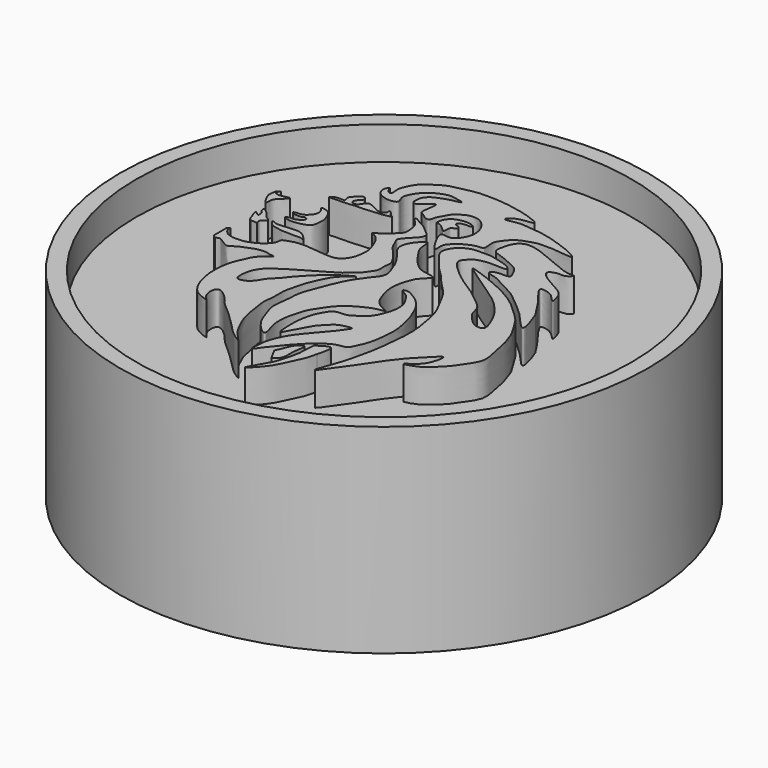
from build123d import *

# Parameters (mm, degrees)
F2_DEPTH  = 60
F3_DEPTH  = 60
F4_DEPTH  = 60
F5_DEPTH  = 60
F6_DEPTH  = 60
F7_DEPTH  = 60
F8_DEPTH  = 60
F9_DEPTH  = 60
F10_DEPTH = 60
F11_DEPTH = 60
F12_DEPTH = 60
F13_DEPTH = 60
F14_DEPTH = 60
F15_DEPTH = 60
F0_R      = 79.4315961508
F0_R_2    = 74.4995271211
F16_DEPTH = 60
F17_DEPTH = 50


with BuildPart() as f2:
    # F1 (on face) → F2 (new body)
    with BuildSketch(Plane.XY):
        with BuildLine():
            add(Edge.make_bspline(
                [(-25.1488033682, 33.7133072317), (-24.948841088, 33.6554055638), (-25.0295864981, 32.2952375615), (-22.7551749783, 31.1580490492), (-23.6359349734, 34.4213041261), (-22.5255529942, 36.8969572813), (-20.9887534088, 39.776852732), (-17.8746981156, 41.548958663), (-15.5329089333, 43.1787274213), (-11.8665002329, 43.7717071714), (-8.4590988449, 44.7027018137), (-5.1828009069, 44.8521876272), (-1.1768115878, 44.7705176008), (2.9007180169, 44.2375848697), (6.6841887942, 43.4421139413), (9.4047457297, 42.6677786162), (14.0223637788, 40.771432856), (9.0739956565, 40.5525862782), (7.7355092347, 39.919706461), (6.8017821417, 39.7666165392), (4.6771433634, 37.4517705589), (9.651774137, 38.8817918711), (11.9523997047, 38.4619543185), (15.5134078486, 38.296345935), (18.6202369187, 37.6878982564), (22.0817429014, 36.7300285599), (25.2590214422, 35.5792190237), (26.9350094416, 34.9827390019), (32.3387299286, 32.2345342215), (24.6677253907, 33.5041153846), (22.3702142175, 33.3721670882), (19.5913401559, 33.5642682328), (16.7071995749, 32.4909140871), (14.0909788157, 31.5624330143), (12.2081344098, 29.2644722909), (10.637791559, 26.9795601204), (11.7320767906, 23.2935134602), (9.3888992863, 23.5231228188), (7.0847764413, 22.6638178094), (5.3482075138, 21.7027677057), (3.7737492872, 20.2886790383), (2.2671681823, 18.7781311135), (3.3463068001, 13.6622313561), (-3.1131224014, 24.214561915), (1.5503065124, 22.2574979025), (3.4773348505, 23.9136026422), (4.8932640063, 26.3636257711), (5.0026084116, 29.0111614257), (4.2133861234, 31.4635114152), (2.2769755793, 33.8530631132), (0.0664367621, 34.6534500458), (-2.5018393163, 34.3215902544), (-3.9733032439, 33.3281410586), (-5.7722556965, 32.0548275906), (-6.5164486797, 30.1206753267), (-7.555684618, 28.8668602689), (-7.7012016356, 26.433035483), (-9.5703340628, 27.0330031457), (-10.7594975132, 28.2654632566), (-11.9803543994, 28.4486728417), (-11.6099857071, 31.2633726711), (-10.9441012767, 35.0474634302), (-13.8731895497, 32.3257538657), (-14.9203635972, 31.151310017), (-16.622592113, 31.1318908236), (-16.5655615782, 33.0655438441), (-16.2974432814, 34.6589808607), (-14.7196124342, 36.3255933191), (-12.2509273921, 37.1340369864), (-10.6075963058, 37.8476618897), (-6.1226589069, 38.5279588204), (-9.9184187928, 39.2690962757), (-11.7829877097, 39.625900886), (-14.3398408927, 38.8250281602), (-16.4524932331, 37.5812630174), (-18.0683920322, 36.2192233402), (-19.4918002513, 33.9877151645), (-20.4148396915, 31.7160870717), (-18.5406189783, 29.1629240945), (-21.6869946154, 28.5886242761), (-23.8178789386, 29.2487292901), (-25.4085790801, 30.1169536255), (-26.4301310689, 32.4230550039), (-25.3572237428, 33.7736580503), (-25.1488033682, 33.7133072317)],
                knots=[0, 0, 0, 0, 0.0088010468, 0.01825747, 0.0300012191, 0.0431291225, 0.0568876526, 0.0712947967, 0.0843234785, 0.0990386418, 0.1135859474, 0.1274974267, 0.142923044, 0.1587382972, 0.1736292931, 0.1878326308, 0.2009766337, 0.2146363917, 0.2246553918, 0.2324142696, 0.2423432307, 0.2567604877, 0.2697582943, 0.2839242077, 0.29780578, 0.3125802409, 0.3263527799, 0.3380840838, 0.3520524286, 0.3691845538, 0.3824486865, 0.3947658058, 0.4083026863, 0.4210882833, 0.4341529226, 0.4470600717, 0.460318558, 0.4701240818, 0.4824347944, 0.4933370912, 0.5043941458, 0.5160546105, 0.5273804796, 0.5482747699, 0.5600336456, 0.5721435882, 0.5849909532, 0.5973202677, 0.6096733329, 0.6229435032, 0.6346210947, 0.6466958716, 0.6570142102, 0.6682888819, 0.6791909485, 0.6892798089, 0.6999278038, 0.7090859349, 0.7193906789, 0.7266444046, 0.7395084249, 0.7518234496, 0.7643086169, 0.7748137274, 0.7831375363, 0.7928370108, 0.8028110507, 0.8141778144, 0.8262877958, 0.8378671653, 0.8508323451, 0.8622235016, 0.8738485587, 0.8861192779, 0.8982292241, 0.9093881265, 0.9219095693, 0.9337973758, 0.9452912312, 0.9568705946, 0.9687588458, 0.9789672473, 0.9908266826, 1, 1, 1, 1], degree=3))
        make_face()
    extrude(amount=F2_DEPTH)


with BuildPart() as f3:
    # F1 (on face) → F3 (new body)
    with BuildSketch(Plane.XY):
        with BuildLine():
            add(Edge.make_bspline(
                [(-26.945585385, 26.3207778335), (-26.5811278754, 26.1919596539), (-25.9021475482, 25.1956940165), (-27.1545322644, 24.3076704164), (-27.7499431243, 23.494602771), (-27.7574333029, 22.2275042374), (-25.897747523, 22.0822792358), (-25.2380605037, 23.4164596333), (-24.2446991532, 24.791559816), (-22.654971193, 24.0563709455), (-20.8721222009, 23.2639980649), (-19.5544966211, 22.4326581284), (-17.5785439162, 23.2834334669), (-18.3095323689, 24.7421037011), (-16.8497931436, 24.0017664095), (-16.7134374099, 22.9181613345), (-15.0603218715, 22.6683654735), (-17.6513601518, 22.0278243921), (-19.5107603166, 21.9286761464), (-21.411838687, 21.7967317051), (-23.4247126983, 21.4454191784), (-25.8274115732, 21.6250141179), (-27.7736671913, 21.2576014296), (-29.5985925328, 21.1885655512), (-31.475130181, 21.3117028241), (-34.3827292896, 20.8634787724), (-31.7377232386, 22.633539097), (-28.9241161492, 21.7104302415), (-30.2136237715, 23.6000988053), (-29.1775773466, 24.8158836205), (-28.1456552657, 25.9685139895), (-27.3010351747, 26.4464122178), (-26.945585385, 26.3207778335)],
                knots=[0, 0, 0, 0, 0.029621162, 0.0602606581, 0.0878346733, 0.114159912, 0.145918635, 0.178271441, 0.2105854405, 0.2435742709, 0.2818298618, 0.3152731713, 0.3499786591, 0.3751276802, 0.4016893464, 0.4305616795, 0.4548520971, 0.4904756287, 0.5303717086, 0.5667593396, 0.6053166578, 0.6470565607, 0.6849271688, 0.7205384141, 0.7603358376, 0.7959315555, 0.8338938186, 0.873661734, 0.9039971078, 0.9365658208, 0.9711109374, 1, 1, 1, 1], degree=3))
        make_face()
    extrude(amount=F3_DEPTH)


with BuildPart() as f4:
    # F1 (on face) → F4 (new body)
    with BuildSketch(Plane.XY):
        with BuildLine():
            add(Edge.make_bspline(
                [(-41.7717136443, -5.5398973636), (-41.812882174, -5.8481698397), (-41.900913535, -6.5073540721), (-41.1781574572, -7.5221923251), (-40.3650623179, -8.3312059894), (-39.5128472879, -8.6372278935), (-38.2526650737, -9.0186086654), (-37.1477285954, -8.9206808049), (-35.7296906683, -8.9229396647), (-34.5576650094, -8.7253272454), (-33.2534097973, -8.2178484871), (-32.019836988, -7.6898016339), (-30.6539944827, -6.8020483209), (-29.5403590759, -5.7476969367), (-28.5482811, -4.3460828042), (-28.8079652144, -2.7393990339), (-27.0064684474, -2.3854852368), (-25.7897787275, -1.8195429094), (-24.2005614178, -1.5944809385), (-22.5584335536, -1.5454733348), (-21.0198860982, -1.6673648427), (-19.3801408161, -1.8562747679), (-17.8724149763, -1.8866949794), (-16.5955273937, -2.1853103978), (-15.0944833944, -2.2375183906), (-13.6987284549, -2.3214296878), (-12.4195594167, -1.9381450275), (-11.0800652344, -1.0484762075), (-10.0296859586, 0.679056702), (-9.5919889509, 2.0539459798), (-9.3615036071, 3.8522474844), (-9.2287679772, 5.4900772478), (-9.7081055721, 7.3552492356), (-10.3886506746, 9.1952918081), (-11.1059511983, 10.8186935734), (-12.3357157318, 12.3516107548), (-13.5188638139, 12.9202228105), (-14.1151761636, 13.2068060338)],
                knots=[0, 0, 0, 0, 0.0226010476, 0.0483282012, 0.0732757833, 0.0955379345, 0.1220339325, 0.1470203337, 0.1747103132, 0.2004493041, 0.227908869, 0.2552804598, 0.2849714154, 0.3143497788, 0.3446015362, 0.3714995697, 0.4004560514, 0.4283986079, 0.4577769801, 0.4879190496, 0.5171292411, 0.5473299531, 0.5760514088, 0.6028558433, 0.6315773079, 0.6592578181, 0.6858933962, 0.7154604959, 0.7484178018, 0.7768371052, 0.8080658597, 0.8382079398, 0.8705581331, 0.9035154357, 0.9347771966, 0.9671273919, 1, 1, 1, 1], degree=3))
            Line((-41.7717136443, -5.5398973636), (-42.4412414432, -6.312427111))
            Line((-42.4412414432, -6.312427111), (-42.4412414432, -10.8445966616))
            add(Edge.make_bspline(
                [(-42.4412414432, -10.8445966616), (-42.3518233963, -10.9601905606), (-42.2624053495, -11.0757844595), (-42.1685176486, -11.1777507043)],
                knots=[0, 0, 0, 0, 0.0071487722, 0.0071487722, 0.0071487722, 0.0071487722], degree=3))
            Line((-42.1685176486, -11.1777507043), (-41.6172109544, -11.5141225979))
            add(Edge.make_bspline(
                [(-41.6172109544, -11.5141225979), (-41.2739568617, -11.5529146812), (-40.5164359526, -11.1174211196), (-39.939617102, -11.4287726818), (-38.5882424276, -12.1381249694), (-36.8538881302, -13.5066791968), (-35.2969900432, -12.2715700906), (-34.1373228627, -11.5753695582), (-31.8539806603, -10.7248807675), (-30.0471463451, -9.9729712348), (-27.2249383164, -9.7223761824), (-26.1800156346, -10.4058344081), (-23.8508093777, -10.1587301465), (-27.812550286, -12.6035494239), (-29.180312977, -15.5258197947), (-30.5844211722, -18.8364875768), (-31.2745911855, -21.6552347309), (-31.398421323, -25.645852678), (-31.0543413286, -28.5636241287), (-29.9953288887, -32.4181815819), (-28.4499579521, -34.7867259671), (-26.8917633836, -36.4207970984), (-22.4800073499, -38.0152544708), (-24.4379324911, -36.6925787292), (-25.1809842613, -35.069793224), (-25.4038326659, -33.248258278), (-24.5324112909, -30.6659563525), (-20.2835539037, -34.1763577811), (-18.790274815, -36.6676925534), (-16.2776501448, -38.467778442), (-13.3398116362, -41.3645848972), (-10.3799188446, -44.1175352927), (-8.1093470247, -46.9412037763), (-4.7698938059, -49.0398547747), (-4.6388213523, -48.9560291171)],
                knots=[0.0195308088, 0.0195308088, 0.0195308088, 0.0195308088, 0.0395165176, 0.0540412535, 0.0776082575, 0.1044403461, 0.1288503292, 0.1515243185, 0.1804790807, 0.2080591077, 0.2388047116, 0.2611253909, 0.2813945091, 0.3151607814, 0.3515490656, 0.3867193244, 0.419334208, 0.4566014451, 0.4897577827, 0.5273175728, 0.5584787467, 0.5892243548, 0.6233580824, 0.6431699724, 0.6695429055, 0.6957509905, 0.720370143, 0.7602568507, 0.7942585309, 0.8266566241, 0.8652890023, 0.9030538629, 0.9420116676, 0.9771089014, 0.9771089014, 0.9771089014, 0.9771089014], degree=3))
            add(Edge.make_bspline(
                [(-4.6388213523, -48.9560291171), (-4.9352998348, -48.6181442496), (-5.2317783172, -48.2802593821), (-5.6173582561, -47.8744879365)],
                knots=[0, 0, 0, 0, 0.0158560937, 0.0158560937, 0.0158560937, 0.0158560937], degree=3))
            add(Edge.make_bspline(
                [(-5.6173582561, -47.8744879365), (-6.13474356, -47.3300089284), (-7.548026456, -45.9398789902), (-8.9315413686, -43.2228054554), (-10.5436119615, -39.9309888811), (-11.3712116442, -36.3589792043), (-11.8973772942, -33.0674972474), (-12.4014600508, -29.8824723696), (-11.7468911414, -26.7704839257), (-11.993439657, -23.4515833025), (-11.6909591902, -21.3795341391), (-10.9799097981, -18.5794695303), (-10.3069577448, -16.3046017593), (-9.2280499592, -13.8182916861), (-8.0760118861, -11.3256808911), (-6.6203654418, -8.9371992375), (-1.7089230724, -5.342087689), (-6.1912461596, -7.8936037937), (-7.942417065, -8.9973623835), (-9.8992416077, -10.9354922771), (-11.7021927255, -12.2806854067), (-12.845209808, -13.7144930258), (-14.8131809385, -15.5870056396), (-16.1569615177, -17.535083997), (-17.4727506994, -18.9539412911), (-18.7450287181, -19.9461027976), (-19.6581344178, -21.6425690566), (-20.910821323, -23.5140413465), (-22.6155281543, -24.6245194996), (-24.6213957754, -24.7646790892), (-24.9895903234, -23.2788042047), (-24.7939524692, -20.5410899606), (-23.9348150765, -18.4398883996), (-22.3816862999, -16.1984506269), (-19.9266940951, -14.7369965943), (-18.0056654028, -13.4090371178), (-16.0930830842, -12.2615334721), (-14.0016017074, -11.2367777297), (-12.1232802741, -9.9159570246), (-9.2286573318, -8.348466506), (-6.8676607355, -6.9464720931), (-5.3930549939, -5.5967884098), (-3.3064302904, -3.8569690441), (-2.193528738, -2.1649292562), (-1.0010126621, -0.4512955562), (-1.466167431, 1.9274365828), (-0.9268812345, 3.716208247), (-1.643877149, 5.1980681997), (-2.1296237756, 6.0366131533), (-2.4242375512, 6.4600519836)],
                knots=[0.0158560937, 0.0158560937, 0.0158560937, 0.0158560937, 0.0371323817, 0.060218382, 0.0853556994, 0.1105165445, 0.1345271615, 0.1578543777, 0.1813702144, 0.2050197665, 0.2241688148, 0.2461795058, 0.2666340445, 0.2881199778, 0.3093962662, 0.3334182674, 0.3586284508, 0.3808198369, 0.4019889386, 0.4232652291, 0.4428666193, 0.4605902908, 0.4821473833, 0.5025765464, 0.5206506722, 0.5370825703, 0.5551800108, 0.5748542534, 0.5936898225, 0.6105447794, 0.6250713915, 0.6467937641, 0.6667689254, 0.6881306205, 0.7102713498, 0.7303665647, 0.7499154225, 0.7697456307, 0.7897207953, 0.8136498657, 0.8353414112, 0.8539609946, 0.875377061, 0.8942214699, 0.9125919059, 0.9325794234, 0.9502390418, 0.966485755, 0.9825739497, 0.9825739497, 0.9825739497, 0.9825739497], degree=3))
            add(Edge.make_bspline(
                [(-3.1750648823, 7.4446975933), (-2.9115332904, 7.1126724104), (-2.6678854208, 6.786362197), (-2.4242375512, 6.4600519836)],
                knots=[0.9672997896, 0.9672997896, 0.9672997896, 0.9672997896, 1, 1, 1, 1], degree=3))
            add(Edge.make_bspline(
                [(-3.1750648823, 7.4446975933), (-3.2842875071, 7.5798804629), (-3.3950326538, 7.7152422973), (-3.5057778005, 7.8506041318)],
                knots=[0.9949376131, 0.9949376131, 0.9949376131, 0.9949376131, 1, 1, 1, 1], degree=3))
            add(Edge.make_bspline(
                [(-10.8190523461, 15.4728898779), (-10.3854274198, 15.9336787565), (-9.5163377594, 16.8572115744), (-7.9802574199, 18.2941033182), (-8.3260002082, 20.4083149948), (-8.4757768683, 22.1852635368), (-9.7512213256, 24.0889997591), (-10.895274758, 24.7182313128), (-10.7579373208, 25.8043581105), (-9.0650849821, 24.457150277), (-7.5303322035, 23.8564050674), (-6.0899522703, 22.7885843373), (-4.9157662853, 21.7113410883), (-3.0425480104, 20.3796482699), (-4.1710010675, 18.0976920702), (-5.8586829505, 16.777319173), (-6.6032379897, 15.7692465224), (-7.4062633733, 14.791681699), (-7.6077682259, 14.1723810275), (-7.1992699425, 13.2583242463), (-6.5296983611, 11.9137837642), (-5.8845376145, 10.4732748357), (-4.8420733277, 9.3388785602), (-3.9296511659, 8.3564771008), (-3.5057778005, 7.8506041318)],
                knots=[0, 0, 0, 0, 0.0480714388, 0.0963468378, 0.1447484497, 0.1916578957, 0.2433048134, 0.2818038524, 0.3068780104, 0.3517429601, 0.3990073719, 0.4441227469, 0.4889877125, 0.537093329, 0.5876362656, 0.6387792572, 0.6779119067, 0.7160563974, 0.7425690758, 0.775907016, 0.8188890711, 0.8621906045, 0.9050766017, 0.9540786737, 0.9540786737, 0.9540786737, 0.9540786737], degree=3))
            Line((-10.8190523461, 15.4728898779), (-12.4156121165, 14.3913496286))
            Line((-12.4156121165, 14.3913496286), (-14.1151761636, 13.2068060338))
        make_face()
    extrude(amount=F4_DEPTH)


with BuildPart() as f5:
    # F1 (on face) → F5 (new body)
    with BuildSketch(Plane.XY):
        with BuildLine():
            add(Edge.make_bspline(
                [(-1.0437119054, 17.6707785577), (-0.6680510269, 17.5281639166), (-0.7167650455, 15.2486465781), (-0.1383137822, 13.1744180567), (1.4633481849, 10.8526251062), (3.1842207352, 8.5119758865), (4.9045450056, 6.7976612166), (7.1274400052, 5.2019533428), (12.4785569794, 5.0404475679), (8.8068904067, 2.095643908), (7.8800533811, 0.092999726), (6.9423578386, -2.7867882957), (6.6287030782, -5.4702540952), (6.9569071786, -8.0680856615), (7.8153266384, -10.6998051683), (8.756228694, -13.1108677491), (11.0125471571, -14.939419708), (14.0214915667, -15.8635478322), (10.7524809013, -16.2119972845), (8.7107193825, -17.0039249448), (6.2489918759, -18.2535355851), (3.5314768148, -20.0089368628), (1.3909330893, -22.3069682992), (0.0560761569, -24.6098040978), (-1.5814909932, -26.726094315), (-2.3159028616, -29.5048403305), (-3.1679217561, -32.3136394185), (-3.3420829586, -35.1384357614), (-3.3290705866, -37.5730381049), (-0.8084833727, -44.3143001347), (-6.596131401, -38.7794677774), (-7.6332647839, -35.1666610179), (-9.5971218339, -30.6324477031), (-8.4865291526, -25.8276229918), (-8.6196646513, -21.382188177), (-6.8158572369, -17.0904387558), (-5.3665305092, -13.0669644448), (-3.1739157096, -8.2219797981), (-0.1030258548, -4.2247765634), (2.1151935011, -1.6009824249), (0.9362872124, 1.8692482935), (0.0377103781, 3.9900265033), (-0.9832666615, 6.0099020432), (-2.4965594418, 8.0176422967), (-3.9154209394, 9.6410443313), (-5.0477323701, 11.748995492), (-4.2503586834, 14.4595533475), (-3.0391121083, 16.0744532453), (-1.4262579955, 17.8160070775), (-1.0437119054, 17.6707785577)],
                knots=[0, 0, 0, 0, 0.0180662574, 0.0370243927, 0.0572922299, 0.0781994976, 0.0968854477, 0.1180022755, 0.1410798269, 0.1619870944, 0.1814118083, 0.2022720423, 0.2223951554, 0.2420617116, 0.2623294907, 0.2817267352, 0.3033696958, 0.3200464418, 0.3374137738, 0.3568024159, 0.3768221173, 0.3988895748, 0.4204704133, 0.4403559629, 0.4601258519, 0.4807435185, 0.5018046219, 0.5216767991, 0.5426840016, 0.568043086, 0.5947742813, 0.6206060917, 0.6468109106, 0.6736301198, 0.6993468146, 0.7253083304, 0.7506873126, 0.7789229723, 0.8065436837, 0.8282051818, 0.8504312216, 0.8692606168, 0.8874684285, 0.9067849697, 0.9248299152, 0.9431665618, 0.9627584908, 0.9816026194, 1, 1, 1, 1], degree=3))
        make_face()
    extrude(amount=F5_DEPTH)


with BuildPart() as f6:
    # F1 (on face) → F6 (new body)
    with BuildSketch(Plane.XY):
        with BuildLine():
            add(Edge.make_bspline(
                [(0.4940500367, -50.237737596), (0.2347112404, -50.1195504862), (0.5103066985, -47.4874990383), (0.6769040843, -45.0440917932), (2.1339693914, -41.387622137), (3.7050160139, -38.788399872), (5.5412466048, -36.4827920712), (7.5080406202, -34.059883027), (9.1278798858, -32.2046935016), (10.817283103, -30.3183952304), (11.7871385117, -28.756592706), (12.913744567, -27.2920623088), (10.8645915202, -27.6372803151), (9.1758834595, -28.045283632), (7.7349563595, -28.8341818338), (6.7234678053, -30.0781462797), (4.937185354, -31.5497243064), (4.0600879869, -33.4080920458), (2.9510748569, -35.3481109623), (2.0395521703, -37.0697354357), (0.1941023116, -40.8101834603), (-0.0407907522, -36.3089590013), (-0.0862577122, -32.928061746), (0.2851370233, -30.5971327924), (0.8636496911, -27.907516707), (2.0920215601, -25.5912182347), (3.6020632392, -22.9439175481), (7.1936462029, -23.4366390418), (9.3826788863, -21.8747289588), (11.6009228324, -20.3955708455), (12.9255803466, -18.5621536991), (13.9308463686, -15.8953019128), (14.4420616775, -14.0800720035), (14.5271562157, -11.8264624082), (14.101712928, -9.6678742439), (12.7191991714, -7.8264112035), (12.0383492387, -6.4096361583), (8.8970202336, -5.0291598162), (10.875153716, -4.505029197), (12.2033139347, -5.129919921), (13.6829661571, -6.0354938103), (15.3539093605, -7.1813244889), (17.1367785085, -9.3188485096), (18.1008405424, -11.0387425305), (19.0196753174, -13.1890438649), (19.741040379, -15.0893606472), (20.3382996294, -17.7424175921), (21.0256114221, -20.5509737958), (21.0761135855, -23.1828525784), (20.8751044174, -26.0087300637), (20.614340675, -28.0506451612), (20.2424546588, -30.1395741867), (19.4532606788, -32.5298353778), (18.2661964925, -34.664102346), (17.8276740631, -36.0436387849), (14.7465090721, -36.1943572681), (12.7880443546, -37.3293463405), (10.1399092464, -38.9882995494), (8.8930488795, -40.4857162659), (6.7513341101, -42.4857538759), (5.3258674891, -44.3866293902), (3.956265061, -46.164528699), (2.5469205402, -47.6785213598), (1.6248592215, -49.0790783624), (0.6928079738, -50.3283165086), (0.4940500367, -50.237737596)],
                knots=[0, 0, 0, 0, 0.016092581, 0.0339180945, 0.0542546768, 0.0726261625, 0.0905454831, 0.1089768296, 0.125528269, 0.1420012813, 0.1569421521, 0.1681094906, 0.1804153048, 0.1950621104, 0.2080806766, 0.2212961181, 0.2370405629, 0.2521013168, 0.2673254649, 0.2833442438, 0.300080553, 0.3175782129, 0.3381229247, 0.3540067764, 0.3710886691, 0.388287161, 0.4054284384, 0.4241330749, 0.4411742212, 0.4580394929, 0.4737808842, 0.49126021, 0.5057400352, 0.5212046687, 0.5367470273, 0.552166403, 0.5661436695, 0.582433472, 0.5931432897, 0.6062331914, 0.6198651472, 0.6348545476, 0.6521589106, 0.6670375318, 0.6827840063, 0.6977604311, 0.7149550262, 0.7327651008, 0.7498254562, 0.7673580245, 0.7823521462, 0.7974302904, 0.8142290104, 0.8305224727, 0.8421328097, 0.8594126185, 0.8757644806, 0.8938490556, 0.9086719618, 0.926354973, 0.9426731525, 0.9582899971, 0.973134778, 0.9876666035, 1, 1, 1, 1], degree=3))
        make_face()
    extrude(amount=F6_DEPTH)


with BuildPart() as f7:
    # F1 (on face) → F7 (new body)
    with BuildSketch(Plane.XY):
        with BuildLine():
            add(Edge.make_bspline(
                [(18.8469719142, -49.53160882), (19.0719934178, -49.7806545768), (22.1820032384, -45.1675211505), (24.9498112967, -41.4884438044), (28.2823518318, -36.2176271983), (32.1522982817, -31.1392206388), (35.0094858383, -28.5958512011), (39.1708604148, -23.9237279851), (37.8900953309, -29.5209605135), (36.2269444405, -32.0675609996), (31.2969069001, -35.0225041773), (37.9577931773, -32.9049060194), (39.8493853557, -30.7644924399), (42.5022304615, -28.3358545822), (44.2052156674, -25.5412026302), (47.4071728821, -21.2312810717), (46.1274634213, -16.6364442877), (45.4475723483, -11.749863183), (43.682085657, -6.5668487602), (41.7652391551, -3.4741507812), (39.6282176401, 0.1751620257), (36.822389871, 2.5221662407), (33.673143652, 5.7327524555), (29.3913591405, 8.4482157029), (25.156195807, 10.5358196796), (21.5820066085, 12.0528026369), (13.1661169107, 15.0802421545), (19.0660731609, 11.5092591014), (21.7037620816, 9.3272432684), (27.1985330921, 5.9511986834), (30.89814968, 2.9897342932), (33.9961501286, -0.7728069078), (35.6436677508, -4.0979926535), (37.3656798254, -8.4616665489), (34.6283021517, -8.7676373231), (32.6239250148, -7.5852406186), (31.2234280381, -5.9426974036), (29.4838217628, -3.9510923182), (29.2524809999, -0.8094724846), (26.0012073144, 1.6927222035), (22.8203343946, 4.3843027436), (18.0123310614, 7.2343368085), (14.5365009944, 9.9977470824), (9.7149973199, 14.3819314201), (11.6389380182, 16.4681916567), (12.9552353036, 17.7816594832), (15.0201346783, 18.2623102132), (17.0260002138, 18.6956982605), (23.5203177194, 18.0844792438), (20.4331307224, 20.2287318766), (17.6651520408, 20.909910287), (14.7226763173, 21.7472413513), (11.8052194672, 21.5225727179), (9.3014093082, 21.6154325262), (6.8987181979, 20.4256415602), (5.2647809323, 18.9434437302), (3.7305111876, 15.7010228061), (6.6289901989, 12.6125540069), (8.8156005327, 9.298601563), (11.7182351492, 7.0041244456), (14.4797531628, 3.1693747907), (18.067790695, 0.1613400375), (19.8224203572, -3.5763257464), (22.8492347556, -8.5650387364), (23.7374692041, -13.9485850872), (24.609976637, -18.6264458729), (24.528291617, -23.4322570166), (23.9885820292, -28.2590560778), (23.446831198, -33.2800633714), (22.1636596445, -37.9229475354), (21.7820609301, -41.3542064841), (18.5537031421, -49.2070294259), (18.8469719142, -49.53160882)],
                knots=[0, 0, 0, 0, 0.0154284311, 0.0323573138, 0.0500648858, 0.0679112112, 0.0831526279, 0.0972034724, 0.1102551915, 0.1246952977, 0.1371758065, 0.1520377671, 0.1653430021, 0.1783630905, 0.1915572404, 0.2075437404, 0.2226706924, 0.2387780105, 0.2553658997, 0.2691293972, 0.2835812948, 0.2972431359, 0.3123542472, 0.3285612449, 0.3436932534, 0.3594025029, 0.3763821589, 0.3900377325, 0.4048183161, 0.4225952803, 0.4384816937, 0.4538957926, 0.4684037771, 0.4822240353, 0.4918099048, 0.5027240925, 0.5132565902, 0.5246458166, 0.5368827435, 0.550908259, 0.5657881969, 0.5823957212, 0.5983693444, 0.6152724437, 0.6255622938, 0.6353924889, 0.6452112731, 0.6566597958, 0.6721487313, 0.6818639569, 0.694735138, 0.7071617154, 0.7193268082, 0.7306219465, 0.7420160056, 0.752745552, 0.7652098764, 0.7792796245, 0.7936538272, 0.807301657, 0.8228386421, 0.8381623151, 0.8526245498, 0.8698046014, 0.8865364521, 0.9021037081, 0.9176819809, 0.9334847207, 0.9496973721, 0.9647836761, 0.979892246, 1, 1, 1, 1], degree=3))
        make_face()
    extrude(amount=F7_DEPTH)


with BuildPart() as f8:
    # F1 (on face) → F8 (new body)
    with BuildSketch(Plane.XY):
        with BuildLine():
            add(Edge.make_bspline(
                [(10.9271435067, -39.9931296706), (12.5184241223, -38.9472879149), (15.8009471323, -36.7899062473), (14.7590611641, -40.849683481), (14.2222540453, -42.9413877428)],
                knots=[0, 0, 0, 0, 0.4847736362, 1, 1, 1, 1], degree=3))
            add(Edge.make_bspline(
                [(10.9271435067, -39.9931296706), (10.9023231736, -41.0342740665), (10.8508065563, -43.1952538249), (10.4849553834, -46.6381873854), (9.0924118884, -51.6404795111), (8.0501965506, -53.6280423898), (3.4148855505, -61.1908405175), (8.7959842228, -55.3563999889), (10.2086672648, -53.0563340807), (11.6766764644, -49.8775775908), (13.3904573107, -46.5748678482), (13.9454153453, -44.1506830756), (14.2222540453, -42.9413877428)],
                knots=[0, 0, 0, 0, 0.0903517968, 0.1875324929, 0.2998290507, 0.3902277539, 0.5079314891, 0.6153417282, 0.7098124994, 0.8024437195, 0.9014498025, 1, 1, 1, 1], degree=3))
        make_face()
    extrude(amount=F8_DEPTH)


with BuildPart() as f9:
    # F1 (on face) → F9 (new body)
    with BuildSketch(Plane.XY):
        with BuildLine():
            add(Edge.make_bspline(
                [(7.1117510088, -51.2658767402), (7.6545782942, -50.8629127925), (8.7366697364, -50.05962996), (9.3143626448, -47.9651218624), (8.8754641497, -45.2667386156), (10.2592459537, -40.5686658048), (6.9777213692, -42.9193336391), (6.3440442839, -45.421277968), (5.5772985706, -46.9805111166), (5.2040554583, -47.7395281196)],
                knots=[0, 0, 0, 0, 0.1254672787, 0.2501109879, 0.4083132923, 0.5710366016, 0.7071200236, 0.857429351, 1, 1, 1, 1], degree=3))
            Line((5.2040554583, -47.7395281196), (7.1117510088, -51.2658767402))
        make_face()
    extrude(amount=F9_DEPTH)


with BuildPart() as f10:
    # F1 (on face) → F10 (new body)
    with BuildSketch(Plane.XY):
        with BuildLine():
            add(Edge.make_bspline(
                [(-31.4861834049, 15.7587900758), (-31.5759823818, 15.6118638231), (-30.79941485, 14.9140694565), (-30.3727654897, 13.9926087382), (-30.4154143053, 13.2584727133), (-30.6098150818, 12.2179853039), (-31.3314528041, 11.5234377386), (-31.8224715842, 10.7800885518), (-33.1304939599, 10.1930750641), (-34.152079337, 10.2618399416), (-35.7289554747, 9.9322818776), (-34.4641956519, 9.2467718038), (-33.5095970152, 9.2281297584), (-32.2867779063, 9.1214282455), (-31.5712395107, 9.8346093035), (-30.5024696149, 9.1775369099), (-30.748730721, 8.4259791261), (-31.656195028, 7.7679527372), (-33.0248260377, 7.0703790325), (-34.1813670012, 7.4619656113), (-35.5518656112, 6.6543599242), (-34.2934846772, 6.2581835834), (-32.7322832935, 5.9465531681), (-30.7183164114, 6.2609234504), (-28.8218630005, 6.7044202266), (-27.3171139766, 7.7703211707), (-27.2920349986, 9.4193861021), (-26.9903761949, 11.3276526021), (-27.5965299708, 12.777464978), (-28.1954108431, 14.272467911), (-29.3590579455, 15.6405045875), (-31.363965785, 15.9587586894), (-31.4861834049, 15.7587900758)],
                knots=[0, 0, 0, 0, 0.0297113266, 0.0610493523, 0.0862312126, 0.1164205144, 0.1459019463, 0.1740941202, 0.2084567041, 0.2413162573, 0.2717665383, 0.2995576028, 0.3309976102, 0.3630540712, 0.3911509081, 0.4203841521, 0.4437379248, 0.4754685834, 0.5117414545, 0.5452708252, 0.5756303936, 0.6024886166, 0.641664581, 0.6843144802, 0.7264918675, 0.7648621025, 0.8021948842, 0.843547735, 0.8806134367, 0.9179943702, 0.9595624834, 1, 1, 1, 1], degree=3))
        make_face()
    extrude(amount=F10_DEPTH)


with BuildPart() as f11:
    # F1 (on face) → F11 (new body)
    with BuildSketch(Plane.XY):
        with BuildLine():
            add(Edge.make_bspline(
                [(-44.0419688821, 16.368214041), (-44.0474841029, 16.424146657), (-44.7609867627, 15.9447441113), (-45.0799864737, 15.4089406691), (-45.243709492, 14.2780405544), (-45.3665635445, 13.2562600458), (-44.8869474236, 12.1427661002), (-44.6031998588, 11.4911866606), (-43.1932955061, 9.0931997759), (-43.1361128154, 10.6230270288), (-43.2056795038, 11.4124557877), (-42.8111420605, 12.2858205783), (-42.3245007432, 12.87806605), (-41.7150023774, 13.4820409751), (-41.1190168508, 13.8438687635), (-40.8430500091, 14.4467130017), (-39.8854828782, 15.1624469282), (-41.2243466108, 15.0178182472), (-42.1021515056, 14.7491191765), (-43.3529566282, 14.5382259461), (-44.2364614946, 14.7980531112), (-45.0532860233, 15.2966460716), (-44.0347551067, 16.2950555325), (-44.0419688821, 16.368214041)],
                knots=[0, 0, 0, 0, 0.041186125, 0.0837173187, 0.1351462678, 0.1860837788, 0.2375224576, 0.2856962306, 0.3553821942, 0.3988275644, 0.4463692659, 0.4930130755, 0.5367058855, 0.5822404606, 0.6223519232, 0.6646792967, 0.7068701433, 0.7517234337, 0.8033348098, 0.857675504, 0.9060266167, 0.9461295449, 1, 1, 1, 1], degree=3))
        make_face()
    extrude(amount=F11_DEPTH)


with BuildPart() as f12:
    # F1 (on face) → F12 (new body)
    with BuildSketch(Plane.XY):
        with BuildLine():
            Line((-40.5653752387, 0.5335501046), (-38.5018847883, 0.3714756167))
            add(Edge.make_bspline(
                [(-38.5018847883, 0.3714756167), (-38.5327005102, 0.520637011), (-38.5983048527, 0.8381903433), (-38.7674243005, 1.4708310845), (-38.617744571, 1.7459340772), (-38.3692407103, 2.0912364817), (-37.9314490014, 2.4158264954), (-36.9564980841, 3.0507527476), (-38.1160675037, 3.7283551949), (-38.8910003209, 4.270416645), (-39.5349852274, 5.3435032996), (-40.2015723412, 6.0565778491), (-40.9414152841, 6.5248978306), (-41.7435403594, 7.3689966204), (-41.7495017284, 5.8127483018), (-40.7469003387, 5.3213794614), (-40.8175417859, 4.2427247165), (-40.5967456313, 3.4197020679), (-41.5911528233, 4.1431797334), (-42.2589226664, 4.7846825267), (-42.1768148732, 3.6059718953), (-41.7327854217, 2.768480731), (-41.4491487726, 2.0607382575), (-41.2067531698, 1.0203134354), (-40.7692566878, 0.6882826085), (-40.5653752387, 0.5335501046)],
                knots=[0, 0, 0, 0, 0.0342475272, 0.0729103964, 0.0993682573, 0.1299400484, 0.1681526624, 0.2126740754, 0.2608511556, 0.3108596717, 0.3646098667, 0.4125950875, 0.4607405807, 0.5019450624, 0.5503232479, 0.6003205177, 0.6503326618, 0.6845759583, 0.7322681427, 0.7716100505, 0.8150144776, 0.8646615494, 0.9075708081, 0.9569262877, 1, 1, 1, 1], degree=3))
        make_face()
    extrude(amount=F12_DEPTH)


with BuildPart() as f13:
    # F1 (on face) → F13 (new body)
    with BuildSketch(Plane.XY):
        with BuildLine():
            add(Edge.make_bspline(
                [(-36.1724644899, 3.3190429676), (-36.1044100287, 3.4608933082), (-34.9332309581, 2.8144857174), (-33.6255644538, 2.8092829529), (-32.119794366, 2.995036459), (-30.5104220523, 2.9579475657), (-28.9213725113, 3.262059871), (-27.7641924258, 3.1005487707), (-26.5387503759, 2.4917151145), (-25.7773310297, 1.7778302718), (-25.2375014524, 1.2237177743), (-24.1081016589, 0.1541045588), (-26.0093205422, 0.9943966541), (-27.052948609, 0.7422322923), (-28.750985331, 0.8499276179), (-30.0390247069, 0.9250698369), (-31.2596527986, 0.8228241351), (-32.7113013121, 1.1495779049), (-34.0095720812, 1.4626123959), (-35.0031527009, 1.5037143674), (-36.2605231812, 3.1354965092), (-36.1724644899, 3.3190429676)],
                knots=[0, 0, 0, 0, 0.0491147433, 0.1051400747, 0.1610705449, 0.2199624616, 0.2780020591, 0.3275094725, 0.3808094485, 0.4269475752, 0.4712068093, 0.5136651527, 0.5660686552, 0.6176350889, 0.6765107173, 0.7291934608, 0.7796115905, 0.8359370279, 0.8880845161, 0.9364482513, 1, 1, 1, 1], degree=3))
        make_face()
    extrude(amount=F13_DEPTH)


with BuildPart() as f14:
    # F1 (on face) → F14 (new body)
    with BuildSketch(Plane.XY):
        with BuildLine():
            add(Edge.make_bspline(
                [(14.2801599577, 26.5449956059), (14.4576997253, 27.3012161962), (14.8014456807, 28.7653826348), (15.9049990116, 30.5684825814), (18.0360365526, 31.7161839429), (21.9968976076, 30.8506129597), (24.4970741864, 29.7858293852), (27.1406804384, 28.6811349344), (30.5043336484, 27.3776746661), (32.4512200068, 26.4429518764), (35.0508887902, 25.7394829222), (36.7747322386, 26.1017495362), (35.940725446, 24.9245474316), (34.5917988718, 24.2493298564), (33.1608016571, 24.489706032), (31.6932973542, 24.2254895578), (29.72275428, 23.2583559455), (32.1616186946, 20.9800539742), (33.669020857, 20.1752565501), (35.4031694495, 19.076620662), (37.5374305306, 18.109350709), (39.6999421899, 16.3757671177), (40.1462866249, 14.8433737519), (41.1426770366, 11.740467395), (38.7427564688, 14.4595082823), (37.8533043198, 15.2777573462), (33.3162368051, 16.5719736646), (36.1827065472, 12.5697102915), (37.722998118, 10.9950813722), (39.471069865, 8.1827330307), (40.9820005505, 5.8808458588), (41.7994968593, 4.6353987418)],
                knots=[0, 0, 0, 0, 0.0345264129, 0.0668487684, 0.1009033016, 0.1460856034, 0.1841595463, 0.2228869116, 0.2659249204, 0.300207145, 0.3382606312, 0.36282611, 0.3842730569, 0.4127090692, 0.439602413, 0.4683685845, 0.496150228, 0.5329015831, 0.5645731105, 0.596400754, 0.6320021506, 0.6686987862, 0.7000871477, 0.7314090615, 0.7650415273, 0.7961929461, 0.8348145721, 0.8750281783, 0.9120374984, 0.9524074657, 1, 1, 1, 1], degree=3))
            add(Edge.make_bspline(
                [(41.7994968593, 4.6353987418), (42.2362950201, 3.5154430871), (43.0646277218, 1.3915882346), (44.6203354357, -4.5401769334), (39.3152350094, 2.0460089261), (38.0012535602, 3.1566093176), (35.4813794697, 5.5475213866), (33.1236923739, 7.2851507209), (31.0791148, 9.1895389296), (28.5948566628, 10.632467065), (25.139805287, 12.2171775295), (22.954706721, 13.7866204199), (18.9377979658, 14.392251289), (21.0941085612, 16.2774388804), (25.6530709852, 15.4461356096), (24.4827242403, 17.7888484723), (23.7346703483, 19.4994153462), (22.1806606967, 20.7608622647), (20.3752933404, 21.3464320839), (18.4344345213, 22.4020583101), (16.2807416156, 23.1158492827), (13.6782236103, 23.9067148804), (14.1425686426, 25.9497877569), (14.2801599577, 26.5449956059)],
                knots=[0, 0, 0, 0, 0.0564028319, 0.1069608673, 0.173877791, 0.2172141754, 0.2675030892, 0.3165959409, 0.3629199187, 0.4108894967, 0.465006317, 0.5141658742, 0.562173667, 0.5982523632, 0.652968289, 0.687787391, 0.7280237728, 0.7666904786, 0.8053847384, 0.846866848, 0.8904276396, 0.9329290141, 0.9751949986, 0.9751949986, 0.9751949986, 0.9751949986], degree=3))
        make_face()
    extrude(amount=F14_DEPTH)


with BuildPart() as f15:
    # F1 (on face) → F15 (new body)
    with BuildSketch(Plane.XY):
        with BuildLine():
            add(Edge.make_bspline(
                [(-5.6183380075, 26.8423389643), (-5.4471559065, 26.6133814972), (-4.1366116905, 27.1077573479), (-1.3652219669, 23.4307791087), (-1.6710745458, 25.8083969459), (-1.2693614049, 27.1578781939), (0.1908919772, 27.0990946788), (0.0011610873, 28.5011665343), (-1.1747133108, 28.6407182387), (-1.5296575024, 28.8579706868), (-1.80001476, 29.6099426933), (-0.8224975979, 29.9986049799), (0.2490108717, 30.2493485905), (1.2619882616, 30.141598775), (2.7885561733, 30.3028853969), (1.359340336, 31.2953490906), (-0.0008541851, 31.3984949539), (-1.1383047659, 31.406916409), (-2.8967333762, 31.0088080263), (-4.1203156288, 30.4496073801), (-5.0859087001, 29.3384884285), (-5.4421033041, 28.3898292277), (-5.7957428697, 27.0796194258), (-5.6183380075, 26.8423389643)],
                knots=[0, 0, 0, 0, 0.0502358166, 0.1291709401, 0.177269734, 0.228184622, 0.2729636701, 0.3148984035, 0.3596774514, 0.3877216935, 0.4210711719, 0.4618732624, 0.5078917994, 0.5545968063, 0.5970088619, 0.6427806613, 0.6954598326, 0.7418655044, 0.7995377745, 0.8505319432, 0.9010969424, 0.9479380258, 1, 1, 1, 1], degree=3))
        make_face()
    extrude(amount=F15_DEPTH)


with BuildPart() as f16:
    # F0 (on Top) → F16 (new body)
    with BuildSketch(Plane.XY):
        Circle(F0_R)
        Circle(F0_R_2, mode=Mode.SUBTRACT)
    extrude(amount=F16_DEPTH)


with BuildPart() as f17:
    # F0 (on Top) → F17 (new body)
    with BuildSketch(Plane.XY):
        Circle(F0_R_2)
    extrude(amount=F17_DEPTH)


solid = Compound([f2.part, f3.part, f4.part, f5.part, f6.part, f7.part, f8.part, f9.part, f10.part, f11.part, f12.part, f13.part, f14.part, f15.part, f16.part, f17.part])
